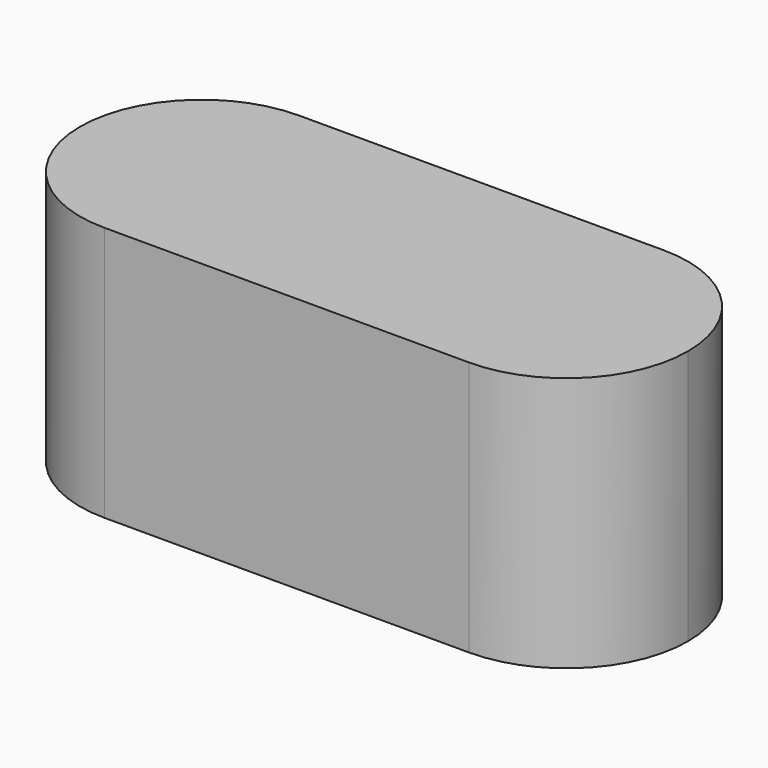
from build123d import *

# Parameters (mm, degrees)
F0_W     = 5
F0_H     = 2
F1_DEPTH = 2.1
F2_R     = 0.99999


# Not quite as in the source:
# - a fillet or chamfer is up to 0.001 mm smaller than in the source, because OpenCascade refuses the exact size


with BuildPart() as f1:
    # F0 (on Top) → F1 (new body)
    with BuildSketch(Plane.XY):
        Rectangle(F0_W, F0_H)
    extrude(amount=F1_DEPTH)

    # F2 (radius 1 in the source; OpenCascade refuses exactly that, so slightly less here)
    f2_edges = [f1.edges().sort_by_distance(p)[0] for p in [
        (2.5, 1, 1.05),
        (2.5, -1, 1.05),
        (-2.5, -1, 1.05),
        (-2.5, 1, 1.05),
    ]]
    fillet(f2_edges, radius=F2_R)


solid = f1.part
